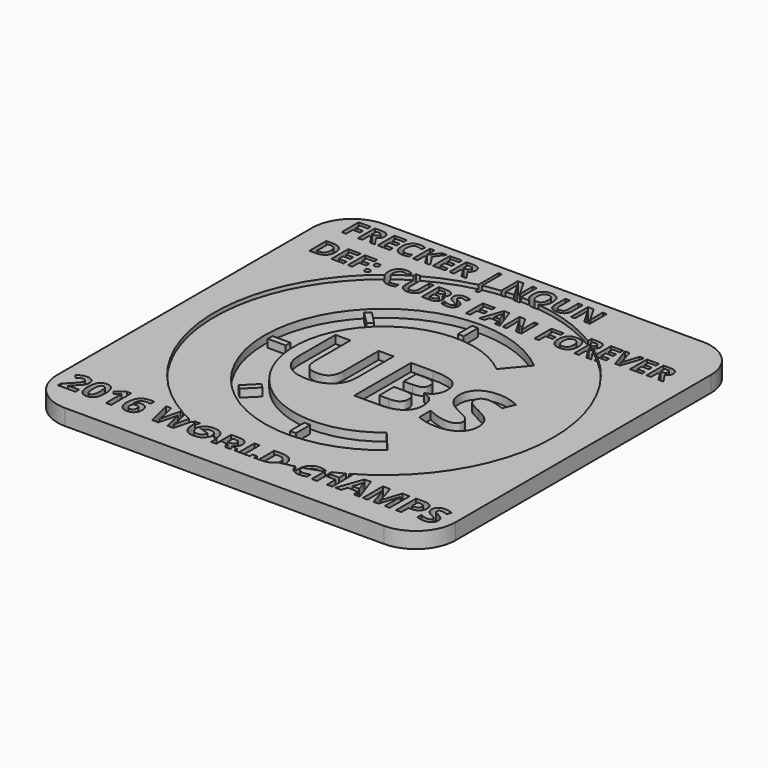
from build123d import *

# Parameters (mm, degrees)
F0_W           = 100
F0_H           = 100
F1_DEPTH       = 2
F3_TEXT_SIZE   = 24.9512670565
F3_TEXT_SIZE_2 = 7.4494639231
F3_TEXT_SIZE_3 = 8.8205425794
F4_DEPTH       = 5
F6_R           = 42.5
F7_DEPTH       = 1
F8_R           = 10
F9_W           = 1.5
F9_H           = 4.5
F9_W_2         = 4.5
F9_H_2         = 1.5
F10_DEPTH      = 2


# Not quite as in the source:
# - Text() gives the source's letters only with a copy of the font that has no kerning and outlines rounded to 1/6400 em; it was checked with that copy


with BuildPart() as f1:
    # F0 (on Top) → F1 (new body, symmetric)
    with BuildSketch(Plane.XY):
        Rectangle(F0_W, F0_H)
    extrude(amount=F1_DEPTH, both=True)

    # F3 (on offset) → F4 (cut)
    with BuildSketch(Plane.XY.offset(-1)):
        with BuildLine():
            Line((14.4627212662, 17.2359999297), (19.2836283302, 22.9813332604))
            ThreePointArc((19.2836283302, 22.9813332604), (-30, 0), (19.2836283302, -22.9813332604))
            Line((19.2836283302, -22.9813332604), (14.4627212476, -17.2359999453))
            ThreePointArc((14.4627212476, -17.2359999453), (-22.5, 1.21e-08), (14.4627212662, 17.2359999297))
        make_face()
        with Locations((-21.3763125771, -8.9824561404)):
            Text('UBS', F3_TEXT_SIZE, font='Open Sans', font_style=FontStyle.BOLD, text_align=(TextAlign.LEFT, TextAlign.BOTTOM))
        with Locations((-45, 42.1363859753)):
            Text('FRECKER | NOUN', F3_TEXT_SIZE_2, font='Open Sans', font_style=FontStyle.BOLD, text_align=(TextAlign.LEFT, TextAlign.BOTTOM))
        with Locations((-45, 32.0051150399)):
            Text('DEF: CUBS FAN FOREVER', F3_TEXT_SIZE_2, font='Open Sans', font_style=FontStyle.BOLD, text_align=(TextAlign.LEFT, TextAlign.BOTTOM))
        with Locations((-47.5, -43.333133258)):
            Text('2016 WORLD CHAMPS', F3_TEXT_SIZE_3, font='Open Sans', font_style=FontStyle.BOLD, text_align=(TextAlign.LEFT, TextAlign.BOTTOM))
    extrude(amount=F4_DEPTH, mode=Mode.SUBTRACT)

    # F6 (on face) → F7 (cut)
    with BuildSketch(Plane.XY.offset(2)):
        Circle(F6_R)
    extrude(amount=-F7_DEPTH, mode=Mode.SUBTRACT)

    # F8
    f8_edges = [f1.edges().sort_by_distance(p)[0] for p in [
        (-50, -50, 0),
        (-50, 50, 0),
        (50, 50, 0),
        (50, -50, 0),
    ]]
    fillet(f8_edges, radius=F8_R)

    # F9 (on face) → F10 (join)
    with BuildSketch(Plane.XY.offset(-1)):
        with Locations((0, 26.3216437677)):
            Rectangle(F9_W, F9_H)
        Polygon((-20.7335331437, 19.6728729719), (-17.5515526283, 16.4908924566), (-16.4908924566, 17.5515526283), (-19.6728729719, 20.7335331437), align=None)
        with Locations((-26.3216437677, 0)):
            Rectangle(F9_W_2, F9_H_2)
        Polygon((-19.6728729719, -20.7335331437), (-16.4908924566, -17.5515526283), (-17.5515526283, -16.4908924566), (-20.7335331437, -19.6728729719), align=None)
        with Locations((0, -26.3216437677)):
            Rectangle(F9_W, F9_H)
    extrude(amount=F10_DEPTH)


solid = f1.part
